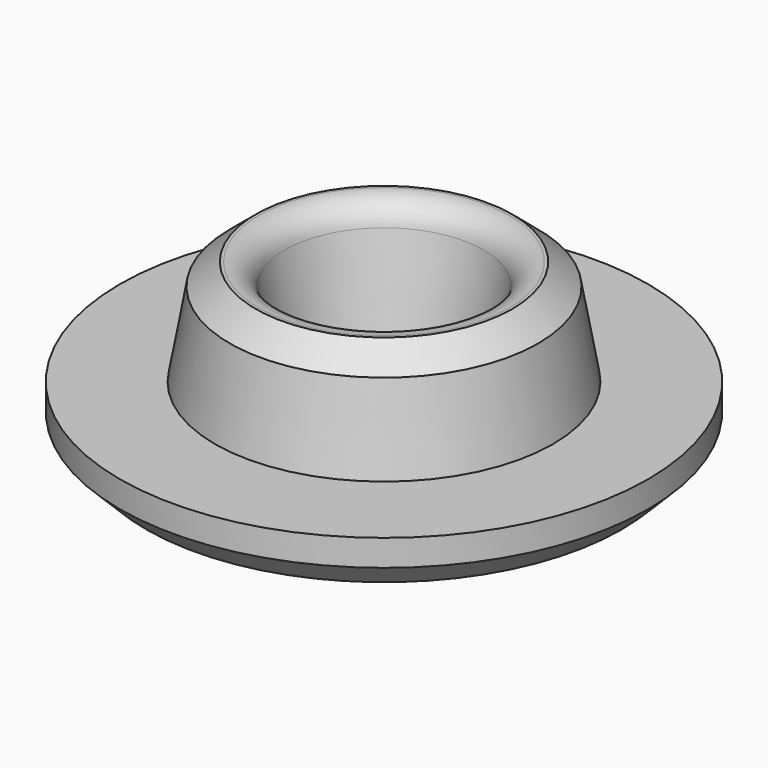
from build123d import *

# Parameters (mm, degrees)
F0_R     = 5
F0_R_2   = 1.6
F1_DEPTH = 1
F2_R     = 3.2
F2_R_2   = 1.6
F3_DEPTH = 2
F3_TAPER = 10
F5_R     = 0.5


# Not quite as in the source:
# - a fillet or chamfer that OpenCascade refuses, or shapes differently, is made with other operations: its cross-section is extruded or revolved along the edge and cut away or added


with BuildPart() as f1:
    # F0 (on Top) → F1 (new body)
    with BuildSketch(Plane.XY):
        Circle(F0_R)
        Circle(F0_R_2, mode=Mode.SUBTRACT)
    extrude(amount=F1_DEPTH)

    # F2 (on face) → F3 (join)
    with BuildSketch(Plane.XY.offset(1)):
        Circle(F2_R)
        Circle(F2_R_2, mode=Mode.SUBTRACT)
    extrude(amount=F3_DEPTH, taper=F3_TAPER)

    # F4: chamfer of 0.5 on 3 edges, made by hand

    # F4_s1 → F4_t2 (revolve, cut)
    with BuildSketch(Plane.XZ):
        Polygon((5, 0.5), (4.5, 0), (5, 0), align=None)
    revolve(axis=Axis((0, 0, 0), (0, 0, 1)), mode=Mode.SUBTRACT)

    # F4_s3 → F4_t4 (revolve, cut)
    with BuildSketch(Plane.XZ):
        Polygon((2.9202000995, 2.5868240888), (2.427796223, 3), (2.8473460386, 3), align=None)
    revolve(axis=Axis((0, 0, 3), (0, 0, -1)), mode=Mode.SUBTRACT)

    # F4_s5 → F4_t6 (revolve, cut)
    with BuildSketch(Plane.XZ):
        Polygon((2.1, 0), (1.6, 0.5), (1.6, 0), align=None)
    revolve(axis=Axis((0, 0, 0), (0, 0, 1)), mode=Mode.SUBTRACT)

    # F5
    f5_edges = [f1.edges().sort_by_distance(p)[0] for p in [
        (-1.952654, 0, 3),
    ]]
    fillet(f5_edges, radius=F5_R)


solid = f1.part
